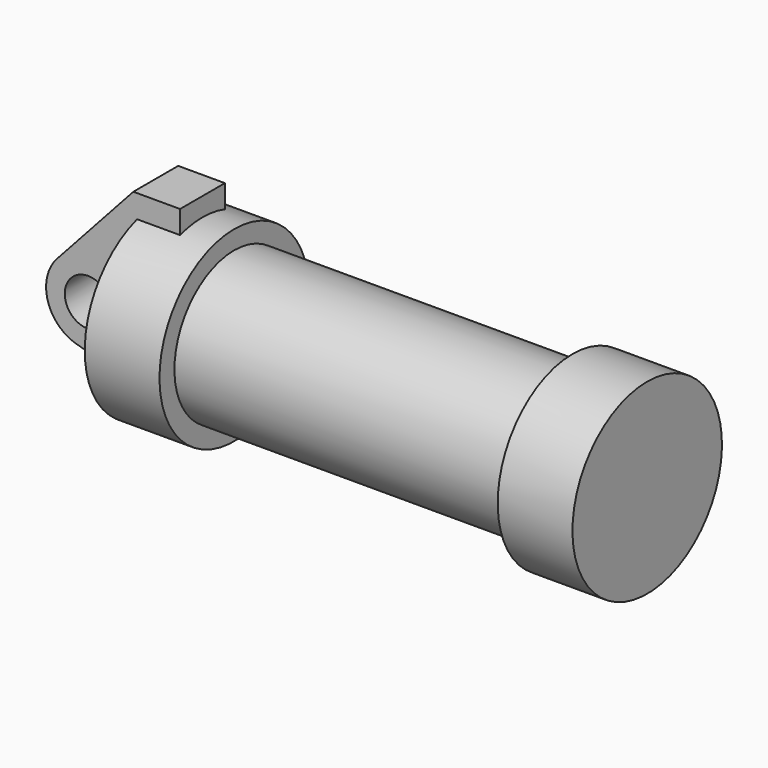
from build123d import *

# Parameters (mm, degrees)
F0_W     = 5.842
F0_H     = 12.7
F0_R     = 3.175
F2_DEPTH = 3.81


# Not quite as in the source:
# - a feature of the source that left no trace in its solid (it failed there, or was rolled back) is left out


with BuildPart() as f1:
    # F0 (on Front) → F1 (revolve)
    with BuildSketch(Plane.XZ):
        Polygon((5.842, 12.7), (5.842, 0), (66.294, 0), (66.294, 12.7), (56.134, 12.7), (56.134, 10.16), (10.16, 10.16), (10.16, 12.7), align=None)
        with Locations((2.921, 6.35)):
            Rectangle(F0_W, F0_H)
    revolve(axis=Axis((33.147, 0, 0), (-1, 0, 0)))

    # F0 (on Front) → F2 (join, symmetric)
    with BuildSketch(Plane.XZ):
        with BuildLine():
            Line((-0.9398, 0), (0, 0))
            Line((0, 0), (0, 12.7))
            Line((0, 12.7), (5.842, 12.7))
            Line((5.842, 12.7), (5.842, 15.24))
            Line((5.842, 15.24), (-0.508, 15.24))
            Line((-0.508, 15.24), (-10.8806298187, 3.8475430269))
            ThreePointArc((-10.8806298187, 3.8475430269), (-4.5919612295, 5.3297205562), (-0.9398, 0))
        make_face()
        with BuildLine():
            ThreePointArc((-8.1826630726, -5.5069827884), (-3.1957909266, -4.5493385486), (-0.9398, 0))
            ThreePointArc((-0.9398, 0), (-4.5919612295, 5.3297205562), (-10.8806298187, 3.8475430269))
            ThreePointArc((-10.8806298187, 3.8475430269), (-12.1459778134, -1.5837270034), (-8.1826630726, -5.5069827884))
        make_face()
        with Locations((-6.6548, 0)):
            Circle(F0_R, mode=Mode.SUBTRACT)
        with BuildLine():
            Line((0, -7.7771894014), (0, 0))
            Line((0, 0), (-0.9398, 0))
            ThreePointArc((-0.9398, 0), (-3.1957909266, -4.5493385486), (-8.1826630726, -5.5069827884))
            Line((-8.1826630726, -5.5069827884), (0, -7.7771894014))
        make_face()
        with Locations((2.921, 6.35)):
            Rectangle(F0_W, F0_H)
        Polygon((5.842, 0), (0, 0), (0, -7.7771894014), (5.842, -9.398), align=None)
    extrude(amount=F2_DEPTH, both=True)


solid = f1.part
